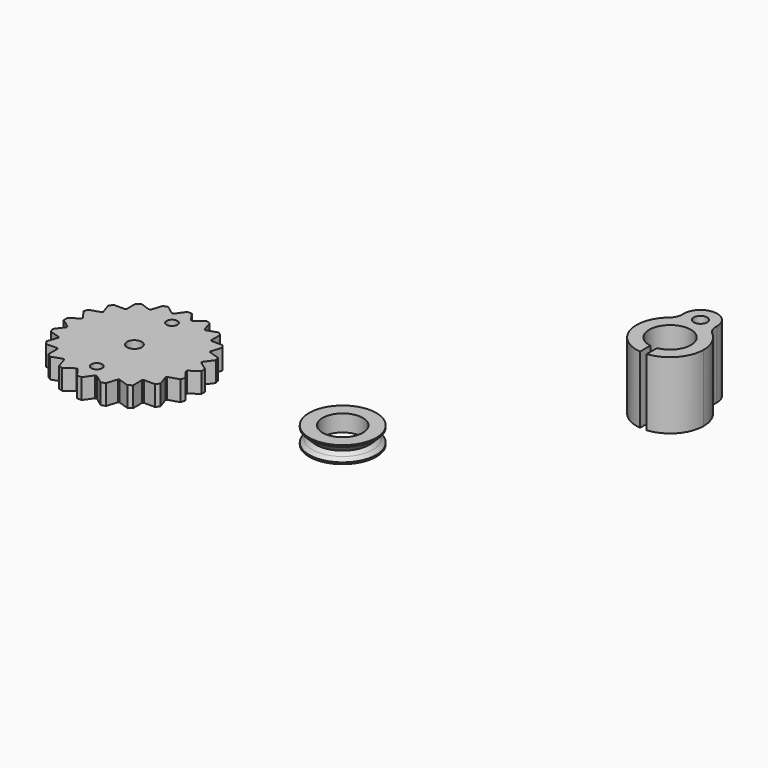
from build123d import *

# Parameters (mm, degrees)
F0_R            = 9
F0_R_2          = 1.1
F1_DEPTH        = 3
F2_R            = 5
F2_R_2          = 3
F3_DEPTH        = 2.5
F5_DEPTH        = 3
F5_COPIES_COUNT = 20
F6_R            = 0.8
F7_DEPTH        = 25
F9_R            = 5
F9_R_2          = 4
F10_DEPTH       = 0.5
F11_SIZE        = 0.49999
F13_DEPTH       = 10
F14_R           = 2


# Not quite as in the source:
# - a fillet or chamfer is up to 0.001 mm smaller than in the source, because OpenCascade refuses the exact size
# - a pattern or mirror of a feature is missing from the dataset's text; its kind, count and spacing are read off the source's solid
# - a feature names something its author has since deleted; it is built from what else it names


with BuildPart() as f1:
    # F0 (on Top) → F1 (new body)
    with BuildSketch(Plane.XY):
        Circle(F0_R)
        Circle(F0_R_2, mode=Mode.SUBTRACT)
    extrude(amount=F1_DEPTH)

    # F4 (on Top) → F5 (join, through all)
    with BuildSketch(Plane.XY):
        with BuildLine():
            Line((1.2998515312, 8.905637877), (0.334630427, 10.2595795691))
            Line((0.334630427, 10.2595795691), (-0.334630427, 10.2595795691))
            Line((-0.334630427, 10.2595795691), (-1.2998515312, 8.905637877))
            ThreePointArc((-1.2998515312, 8.905637877), (0, 9), (1.2998515312, 8.905637877))
        make_face()
    f5 = extrude(amount=F5_DEPTH)

    # F5_copies: F5 ×20 about axis
    f5_copies_axis = Axis((0, 0, 0), (0, 0, 1))
    for i in range(1, F5_COPIES_COUNT):
        add(f5.rotate(f5_copies_axis, i * 360 / F5_COPIES_COUNT))

    # F6 (on Top) → F7 (cut)
    with BuildSketch(Plane.XY):
        with Locations((0, 7)):
            Circle(F6_R)
        with Locations((0, -7)):
            Circle(F6_R)
    extrude(amount=F7_DEPTH, mode=Mode.SUBTRACT)


with BuildPart() as f3:
    # F2 (on Top) → F3 (new body)
    with BuildSketch(Plane.XY):
        with Locations((31.0182180256, 0)):
            Circle(F2_R)
        with Locations((31.0182180256, 0)):
            Circle(F2_R_2, mode=Mode.SUBTRACT)
    extrude(amount=F3_DEPTH)

    # F9 (on mid) → F10 (cut, symmetric)
    with BuildSketch(Plane.XY.offset(1.25)):
        with Locations((31.0182180256, 0)):
            Circle(F9_R)
        with Locations((31.0182180256, 0)):
            Circle(F9_R_2, mode=Mode.SUBTRACT)
    extrude(amount=F10_DEPTH, both=True, mode=Mode.SUBTRACT)

    # F11 (size 0.5 in the source; OpenCascade refuses exactly that, so slightly less here)
    f11_edges = [f3.edges().sort_by_distance(p)[0] for p in [
        (26.018218, 0, 1.75),
        (27.018218, 0, 1.75),
        (26.018218, 0, 0.75),
        (27.018218, 0, 0.75),
    ]]
    chamfer(f11_edges, length=F11_SIZE)


with BuildPart() as f13:
    # F12 (on Top) → F13 (new body)
    with BuildSketch(Plane.XY):
        with BuildLine():
            ThreePointArc((44.6218451609, 49.7635806519), (43.9048883617, 49.4606982518), (43.1879315625, 49.7635806519))
            ThreePointArc((43.1879315625, 49.7635806519), (42.4213351165, 49.5900874785), (41.6913984575, 49.2986042608))
            ThreePointArc((41.6913984575, 49.2986042608), (43.9048883617, 47.9606982518), (46.1183782659, 49.2986042608))
            ThreePointArc((46.1183782659, 49.2986042608), (45.3884416069, 49.5900874785), (44.6218451609, 49.7635806519))
        make_face()
        with BuildLine():
            ThreePointArc((43.1879315625, 49.7635806519), (43.528694794, 51.3872393462), (44.9048883617, 50.4606982518))
            ThreePointArc((44.9048883617, 50.4606982518), (44.8314294561, 50.0845046841), (44.6218451609, 49.7635806519))
            ThreePointArc((44.6218451609, 49.7635806519), (45.3884416069, 49.5900874785), (46.1183782659, 49.2986042608))
            ThreePointArc((46.1183782659, 49.2986042608), (46.3322042415, 49.8622522478), (46.4048883617, 50.4606982518))
            ThreePointArc((46.4048883617, 50.4606982518), (43.3064423576, 52.8880141316), (41.6913984575, 49.2986042608))
            ThreePointArc((41.6913984575, 49.2986042608), (42.4213351165, 49.5900874785), (43.1879315625, 49.7635806519))
        make_face()
        with BuildLine():
            ThreePointArc((46.1183782659, 49.2986042608), (43.9048883617, 47.9606982518), (41.6913984575, 49.2986042608))
            ThreePointArc((41.6913984575, 49.2986042608), (38.9849722484, 43.9239448645), (43.4048883617, 39.8403131472))
            Line((43.4048883617, 39.8403131472), (43.4048883617, 41.7558386246))
            ThreePointArc((43.4048883617, 41.7558386246), (41.8974023717, 47.1774526949), (47.0048883617, 44.8152503327))
            ThreePointArc((47.0048883617, 44.8152503327), (46.2670907239, 42.8077643427), (44.4048883617, 41.7558386246))
            Line((44.4048883617, 41.7558386246), (44.4048883617, 39.8403131472))
            ThreePointArc((44.4048883617, 39.8403131472), (47.6129876052, 41.4611483665), (48.9048883617, 44.8152503327))
            ThreePointArc((48.9048883617, 44.8152503327), (48.15150169, 47.4546205681), (46.1183782659, 49.2986042608))
        make_face()
    extrude(amount=-F13_DEPTH)

    # F14
    f14_edges = [f13.edges().sort_by_distance(p)[0] for p in [
        (46.118378, 49.298604, -5),
        (41.691398, 49.298604, -5),
    ]]
    fillet(f14_edges, radius=F14_R)


solid = Compound([f1.part, f3.part, f13.part])
